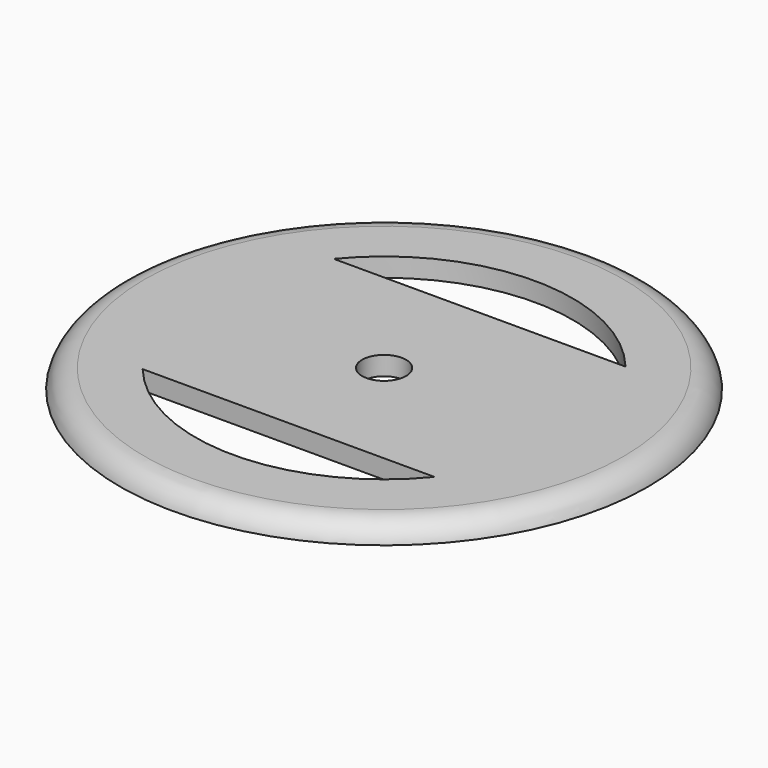
from build123d import *

# Parameters (mm, degrees)
F1_R     = 42
F2_DEPTH = 3
F3_DEPTH = 3
F6_DEPTH = 30


# Not quite as in the source:
# - a fillet or chamfer that OpenCascade refuses, or shapes differently, is made with other operations: its cross-section is extruded or revolved along the edge and cut away or added


with BuildPart() as f2:
    # F1 (on Top) → F2 (new body)
    with BuildSketch(Plane.XY):
        with Locations((9.5, 0)):
            Circle(F1_R)
    extrude(amount=F2_DEPTH)

    # F0 (on Top) → F3 (cut)
    with BuildSketch(Plane.XY):
        with BuildLine():
            Line((6, 0), (13, 0))
            ThreePointArc((13, 0), (9.5, 3.5), (6, 0))
        make_face()
        with BuildLine():
            ThreePointArc((6, 0), (9.5, -3.5), (13, 0))
            Line((13, 0), (6, 0))
        make_face()
    extrude(amount=F3_DEPTH, mode=Mode.SUBTRACT)

    # F4: fillet of radius 4 on 1 edges, made by hand

    # F4_s1 → F4_t2 (revolve, cut)
    with BuildSketch(Plane.XZ):
        with BuildLine():
            ThreePointArc((51.5, 0), (50.0765063966, 2.1622776602), (47.6270166538, 3))
            Line((47.6270166538, 3), (51.5, 3))
            Line((51.5, 3), (51.5, 0))
        make_face()
    revolve(axis=Axis((9.5, 0, 3), (0, 0, 1)), mode=Mode.SUBTRACT)

    # F5 (on face) → F6 (cut)
    with BuildSketch(Plane.XY):
        with BuildLine():
            Line((-13.7163735325, 19), (32.7163735325, 19))
            ThreePointArc((32.7163735325, 19), (9.5, 30), (-13.7163735325, 19))
        make_face()
        with BuildLine():
            Line((32.7163735325, -19), (-13.7163735325, -19))
            ThreePointArc((-13.7163735325, -19), (9.5, -30), (32.7163735325, -19))
        make_face()
    extrude(amount=F6_DEPTH, mode=Mode.SUBTRACT)


solid = f2.part
